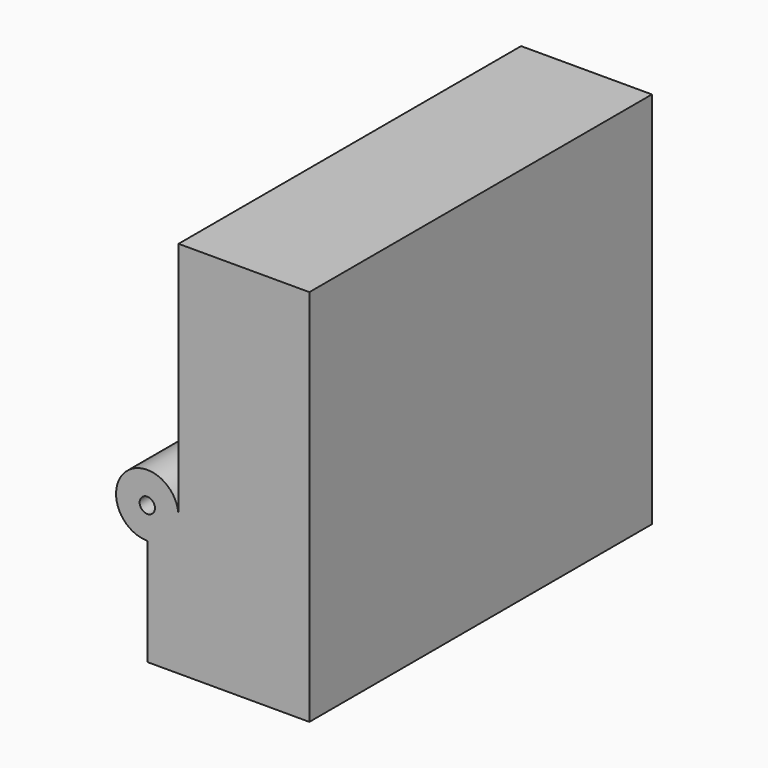
from build123d import *

# Parameters (mm, degrees)
F1_DEPTH      = 25.4
F2_DEPTH      = 25.4
F3_DEPTH      = 99.822
F3_DEPTH_BACK = 25.4
F4_D          = 6.35
F5_DEPTH      = 127


# Not quite as in the source:
# - a feature names something its author has since deleted; it is built from what else it names


with BuildPart() as f1:
    # F0 (on Front) → F1 (new body)
    with BuildSketch(Plane.XZ):
        with BuildLine():
            Line((32.0781692863, 21.0455041379), (-22.2560535658, 21.0455041379))
            ThreePointArc((-22.2560535658, 21.0455041379), (-26.0561402101, 11.8712834228), (-35.2303609252, 8.0711967784))
            Line((-35.2303609252, 8.0711967784), (-35.2303609252, -36.2501852214))
            Line((-35.2303609252, -36.2501852214), (32.0781692863, -36.2501852214))
            Line((32.0781692863, -36.2501852214), (32.0781692863, 21.0455041379))
        make_face()
        with BuildLine():
            Line((-22.2560535658, 21.0455041379), (-35.2303609252, 21.0455041379))
            Line((-35.2303609252, 21.0455041379), (-35.2303609252, 8.0711967784))
            ThreePointArc((-35.2303609252, 8.0711967784), (-26.0561402101, 11.8712834228), (-22.2560535658, 21.0455041379))
        make_face()
        with BuildLine():
            Line((-35.2303609252, 8.0711967784), (-35.2303609252, 21.0455041379))
            Line((-35.2303609252, 21.0455041379), (-22.2560535658, 21.0455041379))
            ThreePointArc((-22.2560535658, 21.0455041379), (-44.4045816403, 30.2197248529), (-35.2303609252, 8.0711967784))
        make_face()
    extrude(amount=F1_DEPTH)

    # F2 (add): a face of the model
    f2_faces = [f1.faces().sort_by_distance(p)[0] for p in [
        (-4.8856962064, -25.4, -4.7596143665),
    ]]
    extrude(f2_faces, amount=F2_DEPTH)

    # F3 (add, two sides): a face of the model
    f3_faces = [f1.faces().sort_by_distance(p)[0] for p in [
        (4.9110578602, -25.4, 21.0455041379),
    ]]
    extrude(f3_faces, amount=F3_DEPTH)
    extrude(f3_faces, amount=-F3_DEPTH_BACK)

    # F4 (through all)
    with Locations(Plane(origin=(0, 0, 0), x_dir=(1, 0, 0), z_dir=(0, 1, 0))):
        with Locations((-35.2303609252, -21.0455041379)):
            Hole(F4_D / 2)

    # F5 (add): a face of the model
    f5_faces = [f1.faces().sort_by_distance(p)[0] for p in [
        (0.7229147363, 0, 37.7328540078),
    ]]
    extrude(f5_faces, amount=F5_DEPTH)


solid = f1.part
